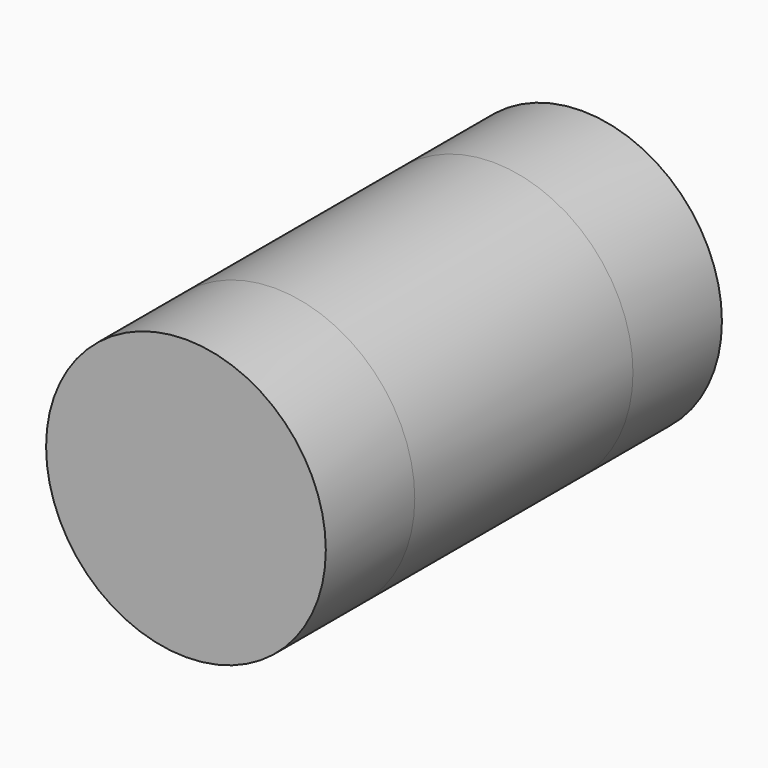
from build123d import *

# Parameters (mm, degrees)
F0_R     = 50.8
F1_DEPTH = 139.446


# Not quite as in the source:
# - a feature of the source that left no trace in its solid (it failed there, or was rolled back) is left out
# - a pattern or mirror of a feature is missing from the dataset's text; its kind, count and spacing are read off the source's solid


with BuildPart() as f1:
    # F0 (on Front) → F1 (new body)
    with BuildSketch(Plane.XZ):
        Circle(F0_R)
    extrude(amount=F1_DEPTH)

    # F1_copies: F1 across plane


with BuildPart() as f1_1:
    add(f1.part)
    add(f1.part.mirror(Plane.ZX.offset(-49.53)))


solid = f1_1.part
